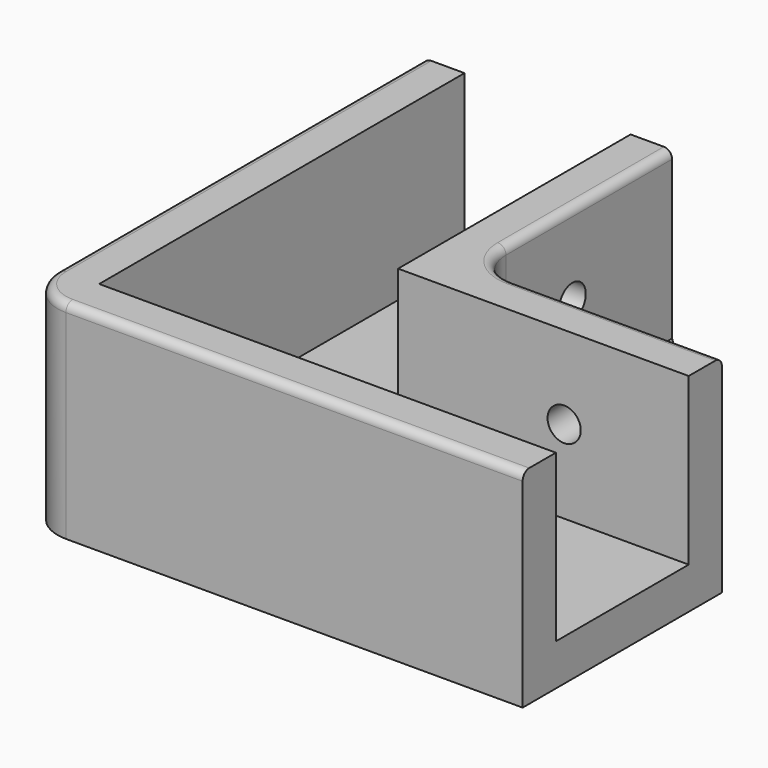
from build123d import *

# Parameters (mm, degrees)
F1_DEPTH  = 5
F3_DEPTH  = 20
F6_R      = 2.4197546063
F7_DEPTH  = 25
F8_R      = 5
F9_R      = 5
F10_R     = 1
F4_R      = 2
F11_DEPTH = 10
F5_R      = 2
F12_DEPTH = 10


with BuildPart() as f1:
    # F0 (on Top) → F1 (new body)
    with BuildSketch(Plane.XY):
        Polygon((-23.4292047727, 30), (-53.4292047727, 30), (-53.4292047727, -30), (6.5707952273, -30), (6.5707952273, 0), align=None)
    extrude(amount=F1_DEPTH)

    # F2 (on face) → F3 (join)
    with BuildSketch(Plane.XY.offset(5)):
        Polygon((6.5707952273, -30), (6.5707952273, -25), (-48.4292047727, -25), (-48.4292047727, 30), (-53.4292047727, 30), (-53.4292047727, -30), align=None)
        Polygon((-28.4292047727, 30), (-28.4292047727, -5), (6.5707952273, -5), (6.5707952273, 0), (-23.4292047727, 0), (-23.4292047727, 30), align=None)
    extrude(amount=F3_DEPTH)

    # F6 (on face) → F7 (cut)
    with BuildSketch(Plane.XY.offset(5)):
        with Locations((-15.4292047727, 8)):
            Circle(F6_R)
    extrude(amount=-F7_DEPTH, mode=Mode.SUBTRACT)

    # F8
    f8_edges = [f1.edges().sort_by_distance(p)[0] for p in [
        (-23.429205, 0, 15),
    ]]
    fillet(f8_edges, radius=F8_R)

    # F9
    f9_edges = [f1.edges().sort_by_distance(p)[0] for p in [
        (-53.429205, -30, 12.5),
    ]]
    fillet(f9_edges, radius=F9_R)

    # F10
    f10_edges = [f1.edges().sort_by_distance(p)[0] for p in [
        (-20.929205, -30, 25),
        (-23.429205, 17.5, 25),
        (-53.429205, 2.5, 25),
        (-51.964739, -28.535534, 25),
        (-5.929205, 0, 25),
        (-21.964739, 1.464466, 25),
    ]]
    fillet(f10_edges, radius=F10_R)

    # F4 (on face) → F11 (cut)
    with BuildSketch(Plane.YZ.offset(-23.4292047727)):
        with Locations((15, 15)):
            Circle(F4_R)
    extrude(amount=-F11_DEPTH, mode=Mode.SUBTRACT)

    # F5 (on face) → F12 (cut)
    with BuildSketch(Plane(origin=(0, 0, 0), x_dir=(-1, 0, 0), z_dir=(0, 1, 0))):
        with Locations((8.4292047727, 15)):
            Circle(F5_R)
    extrude(amount=-F12_DEPTH, mode=Mode.SUBTRACT)


solid = f1.part
